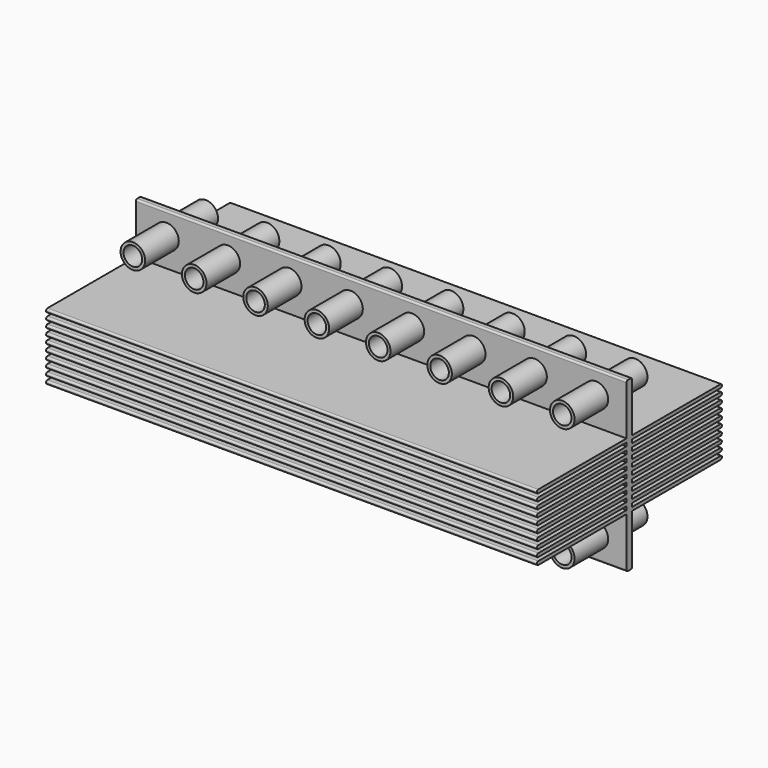
from build123d import *

# Parameters (mm, degrees)
F0_W      = 889
F0_H      = 304.8
F1_DEPTH  = 12.7
F3_D      = 33.655
F5_DEPTH  = 889
F6_R      = 3.175
F7_R      = 22.2377
F7_R_2    = 16.8275
F8_DEPTH  = 76.2
F9_R      = 22.2377
F9_R_2    = 16.8275
F10_DEPTH = 76.2


# Not quite as in the source:
# - after a boolean that leaves OpenCascade's solid faulty, fix() repairs it


with BuildPart() as f1:
    # F0 (on Front) → F1 (new body)
    with BuildSketch(Plane.XZ):
        with Locations((444.5, 152.4)):
            Rectangle(F0_W, F0_H)
    extrude(amount=F1_DEPTH)

    # F3 (through all)
    with Locations(Plane.XZ.offset(12.7)):
        with Locations((55.5752, 41.275), (55.5752, 263.5504), (166.7002, 263.5504), (166.7002, 41.275), (277.8252, 41.275), (277.8252, 263.5504), (388.9502, 263.5504), (500.0752, 41.275), (500.0752, 263.5504), (388.9502, 41.275), (611.2002, 41.275), (722.3252, 41.275), (833.4502, 41.275), (833.4502, 263.5504), (722.3252, 263.5504), (611.2002, 263.5504)):
            Hole(F3_D / 2)

    # F4 (on face) → F5 (join, through all)
    with BuildSketch(Plane(origin=(0, 0, 0), x_dir=(0, -1, 0), z_dir=(-1, 0, 0))):
        with BuildLine():
            Line((212.725, 161.925), (12.7, 161.925))
            Line((12.7, 161.925), (12.7, 155.575))
            Line((12.7, 155.575), (212.725, 155.575))
            ThreePointArc((212.725, 155.575), (214.9700640303, 156.5049359697), (215.9, 158.75))
            ThreePointArc((215.9, 158.75), (214.9700640303, 160.9950640303), (212.725, 161.925))
        make_face()
        with BuildLine():
            Line((212.725, 174.625), (12.7, 174.625))
            Line((12.7, 174.625), (12.7, 168.275))
            Line((12.7, 168.275), (212.725, 168.275))
            ThreePointArc((212.725, 168.275), (214.9700640303, 169.2049359697), (215.9, 171.45))
            ThreePointArc((215.9, 171.45), (214.9700640303, 173.6950640303), (212.725, 174.625))
        make_face()
        with BuildLine():
            Line((212.725, 187.325), (12.7, 187.325))
            Line((12.7, 187.325), (12.7, 180.975))
            Line((12.7, 180.975), (212.725, 180.975))
            ThreePointArc((212.725, 180.975), (214.9700640303, 181.9049359697), (215.9, 184.15))
            ThreePointArc((215.9, 184.15), (214.9700640303, 186.3950640303), (212.725, 187.325))
        make_face()
        with BuildLine():
            Line((212.725, 200.025), (12.7, 200.025))
            Line((12.7, 200.025), (12.7, 193.675))
            Line((12.7, 193.675), (212.725, 193.675))
            ThreePointArc((212.725, 193.675), (214.9700640303, 194.6049359697), (215.9, 196.85))
            ThreePointArc((215.9, 196.85), (214.9700640303, 199.0950640303), (212.725, 200.025))
        make_face()
        with BuildLine():
            Line((212.725, 212.725), (12.7, 212.725))
            Line((12.7, 212.725), (12.7, 206.375))
            Line((12.7, 206.375), (212.725, 206.375))
            ThreePointArc((212.725, 206.375), (214.9700640303, 207.3049359697), (215.9, 209.55))
            ThreePointArc((215.9, 209.55), (214.9700640303, 211.7950640303), (212.725, 212.725))
        make_face()
        with BuildLine():
            Line((12.7, 98.425), (12.7, 92.075))
            Line((12.7, 92.075), (212.725, 92.075))
            ThreePointArc((212.725, 92.075), (214.9700640303, 93.0049359697), (215.9, 95.25))
            ThreePointArc((215.9, 95.25), (214.9700640303, 97.4950640303), (212.725, 98.425))
            Line((212.725, 98.425), (12.7, 98.425))
        make_face()
        with BuildLine():
            Line((12.7, 111.125), (12.7, 104.775))
            Line((12.7, 104.775), (212.725, 104.775))
            ThreePointArc((212.725, 104.775), (214.9700640303, 105.7049359697), (215.9, 107.95))
            ThreePointArc((215.9, 107.95), (214.9700640303, 110.1950640303), (212.725, 111.125))
            Line((212.725, 111.125), (12.7, 111.125))
        make_face()
        with BuildLine():
            Line((12.7, 123.825), (12.7, 117.475))
            Line((12.7, 117.475), (212.725, 117.475))
            ThreePointArc((212.725, 117.475), (214.9700640303, 118.4049359697), (215.9, 120.65))
            ThreePointArc((215.9, 120.65), (214.9700640303, 122.8950640303), (212.725, 123.825))
            Line((212.725, 123.825), (12.7, 123.825))
        make_face()
        with BuildLine():
            Line((12.7, 136.525), (12.7, 130.175))
            Line((12.7, 130.175), (212.725, 130.175))
            ThreePointArc((212.725, 130.175), (214.9700640303, 131.1049359697), (215.9, 133.35))
            ThreePointArc((215.9, 133.35), (214.9700640303, 135.5950640303), (212.725, 136.525))
            Line((212.725, 136.525), (12.7, 136.525))
        make_face()
        with BuildLine():
            Line((12.7, 149.225), (12.7, 142.875))
            Line((12.7, 142.875), (212.725, 142.875))
            ThreePointArc((212.725, 142.875), (214.9700640303, 143.8049359697), (215.9, 146.05))
            ThreePointArc((215.9, 146.05), (214.9700640303, 148.2950640303), (212.725, 149.225))
            Line((212.725, 149.225), (12.7, 149.225))
        make_face()
        with BuildLine():
            Line((0, 206.375), (0, 212.725))
            Line((0, 212.725), (-200.025, 212.725))
            ThreePointArc((-200.025, 212.725), (-202.2700640303, 211.7950640303), (-203.2, 209.55))
            ThreePointArc((-203.2, 209.55), (-202.2700640303, 207.3049359697), (-200.025, 206.375))
            Line((-200.025, 206.375), (0, 206.375))
        make_face()
        with BuildLine():
            Line((0, 193.675), (0, 200.025))
            Line((0, 200.025), (-200.025, 200.025))
            ThreePointArc((-200.025, 200.025), (-202.2700640303, 199.0950640303), (-203.2, 196.85))
            ThreePointArc((-203.2, 196.85), (-202.2700640303, 194.6049359697), (-200.025, 193.675))
            Line((-200.025, 193.675), (0, 193.675))
        make_face()
        with BuildLine():
            Line((0, 180.975), (0, 187.325))
            Line((0, 187.325), (-200.025, 187.325))
            ThreePointArc((-200.025, 187.325), (-202.2700640303, 186.3950640303), (-203.2, 184.15))
            ThreePointArc((-203.2, 184.15), (-202.2700640303, 181.9049359697), (-200.025, 180.975))
            Line((-200.025, 180.975), (0, 180.975))
        make_face()
        with BuildLine():
            Line((0, 168.275), (0, 174.625))
            Line((0, 174.625), (-200.025, 174.625))
            ThreePointArc((-200.025, 174.625), (-202.2700640303, 173.6950640303), (-203.2, 171.45))
            ThreePointArc((-203.2, 171.45), (-202.2700640303, 169.2049359697), (-200.025, 168.275))
            Line((-200.025, 168.275), (0, 168.275))
        make_face()
        with BuildLine():
            Line((0, 155.575), (0, 161.925))
            Line((0, 161.925), (-200.025, 161.925))
            ThreePointArc((-200.025, 161.925), (-202.2700640303, 160.9950640303), (-203.2, 158.75))
            ThreePointArc((-203.2, 158.75), (-202.2700640303, 156.5049359697), (-200.025, 155.575))
            Line((-200.025, 155.575), (0, 155.575))
        make_face()
        with BuildLine():
            Line((-200.025, 142.875), (0, 142.875))
            Line((0, 142.875), (0, 149.225))
            Line((0, 149.225), (-200.025, 149.225))
            ThreePointArc((-200.025, 149.225), (-202.2700640303, 148.2950640303), (-203.2, 146.05))
            ThreePointArc((-203.2, 146.05), (-202.2700640303, 143.8049359697), (-200.025, 142.875))
        make_face()
        with BuildLine():
            Line((-200.025, 130.175), (0, 130.175))
            Line((0, 130.175), (0, 136.525))
            Line((0, 136.525), (-200.025, 136.525))
            ThreePointArc((-200.025, 136.525), (-202.2700640303, 135.5950640303), (-203.2, 133.35))
            ThreePointArc((-203.2, 133.35), (-202.2700640303, 131.1049359697), (-200.025, 130.175))
        make_face()
        with BuildLine():
            Line((-200.025, 117.475), (0, 117.475))
            Line((0, 117.475), (0, 123.825))
            Line((0, 123.825), (-200.025, 123.825))
            ThreePointArc((-200.025, 123.825), (-202.2700640303, 122.8950640303), (-203.2, 120.65))
            ThreePointArc((-203.2, 120.65), (-202.2700640303, 118.4049359697), (-200.025, 117.475))
        make_face()
        with BuildLine():
            Line((-200.025, 104.775), (0, 104.775))
            Line((0, 104.775), (0, 111.125))
            Line((0, 111.125), (-200.025, 111.125))
            ThreePointArc((-200.025, 111.125), (-202.2700640303, 110.1950640303), (-203.2, 107.95))
            ThreePointArc((-203.2, 107.95), (-202.2700640303, 105.7049359697), (-200.025, 104.775))
        make_face()
        with BuildLine():
            Line((-200.025, 92.075), (0, 92.075))
            Line((0, 92.075), (0, 98.425))
            Line((0, 98.425), (-200.025, 98.425))
            ThreePointArc((-200.025, 98.425), (-202.2700640303, 97.4950640303), (-203.2, 95.25))
            ThreePointArc((-203.2, 95.25), (-202.2700640303, 93.0049359697), (-200.025, 92.075))
        make_face()
    extrude(amount=-F5_DEPTH)

    # F6
    f6_edges = [f1.edges().sort_by_distance(p)[0] for p in [
        (444.5, 0, 0),
        (444.5, -12.7, 0),
        (444.5, -12.7, 304.8),
        (444.5, 0, 304.8),
    ]]
    fillet(f6_edges, radius=F6_R)

    # F7 (on face) → F8 (join)
    with BuildSketch(Plane(origin=(0, 0, 0), x_dir=(-1, 0, 0), z_dir=(0, 1, 0))):
        with Locations((-55.5752, 41.275)):
            Circle(F7_R)
        with Locations((-55.5752, 41.275)):
            Circle(F7_R_2, mode=Mode.SUBTRACT)
        with Locations((-55.5752, 263.5504)):
            Circle(F7_R)
        with Locations((-55.5752, 263.5504)):
            Circle(F7_R_2, mode=Mode.SUBTRACT)
        with Locations((-166.7002, 41.275)):
            Circle(F7_R)
        with Locations((-166.7002, 41.275)):
            Circle(F7_R_2, mode=Mode.SUBTRACT)
        with Locations((-166.7002, 263.5504)):
            Circle(F7_R)
        with Locations((-166.7002, 263.5504)):
            Circle(F7_R_2, mode=Mode.SUBTRACT)
        with Locations((-277.8252, 41.275)):
            Circle(F7_R)
        with Locations((-277.8252, 41.275)):
            Circle(F7_R_2, mode=Mode.SUBTRACT)
        with Locations((-277.8252, 263.5504)):
            Circle(F7_R)
        with Locations((-277.8252, 263.5504)):
            Circle(F7_R_2, mode=Mode.SUBTRACT)
        with Locations((-388.9502, 41.275)):
            Circle(F7_R)
        with Locations((-388.9502, 41.275)):
            Circle(F7_R_2, mode=Mode.SUBTRACT)
        with Locations((-388.9502, 263.5504)):
            Circle(F7_R)
        with Locations((-388.9502, 263.5504)):
            Circle(F7_R_2, mode=Mode.SUBTRACT)
        with Locations((-500.0752, 41.275)):
            Circle(F7_R)
        with Locations((-500.0752, 41.275)):
            Circle(F7_R_2, mode=Mode.SUBTRACT)
        with Locations((-500.0752, 263.5504)):
            Circle(F7_R)
        with Locations((-500.0752, 263.5504)):
            Circle(F7_R_2, mode=Mode.SUBTRACT)
        with Locations((-611.2002, 41.275)):
            Circle(F7_R)
        with Locations((-611.2002, 41.275)):
            Circle(F7_R_2, mode=Mode.SUBTRACT)
        with Locations((-611.2002, 263.5504)):
            Circle(F7_R)
        with Locations((-611.2002, 263.5504)):
            Circle(F7_R_2, mode=Mode.SUBTRACT)
        with Locations((-722.3252, 41.275)):
            Circle(F7_R)
        with Locations((-722.3252, 41.275)):
            Circle(F7_R_2, mode=Mode.SUBTRACT)
        with Locations((-722.3252, 263.5504)):
            Circle(F7_R)
        with Locations((-722.3252, 263.5504)):
            Circle(F7_R_2, mode=Mode.SUBTRACT)
        with Locations((-833.4502, 41.275)):
            Circle(F7_R)
        with Locations((-833.4502, 41.275)):
            Circle(F7_R_2, mode=Mode.SUBTRACT)
        with Locations((-833.4502, 263.5504)):
            Circle(F7_R)
        with Locations((-833.4502, 263.5504)):
            Circle(F7_R_2, mode=Mode.SUBTRACT)
    extrude(amount=F8_DEPTH)

    # F9 (on face) → F10 (join)
    with BuildSketch(Plane.XZ.offset(12.7)):
        with Locations((55.5752, 41.275)):
            Circle(F9_R)
        with Locations((55.5752, 41.275)):
            Circle(F9_R_2, mode=Mode.SUBTRACT)
        with Locations((55.5752, 263.5504)):
            Circle(F9_R)
        with Locations((55.5752, 263.5504)):
            Circle(F9_R_2, mode=Mode.SUBTRACT)
        with Locations((166.7002, 41.275)):
            Circle(F9_R)
        with Locations((166.7002, 41.275)):
            Circle(F9_R_2, mode=Mode.SUBTRACT)
        with Locations((166.7002, 263.5504)):
            Circle(F9_R)
        with Locations((166.7002, 263.5504)):
            Circle(F9_R_2, mode=Mode.SUBTRACT)
        with Locations((277.8252, 41.275)):
            Circle(F9_R)
        with Locations((277.8252, 41.275)):
            Circle(F9_R_2, mode=Mode.SUBTRACT)
        with Locations((277.8252, 263.5504)):
            Circle(F9_R)
        with Locations((277.8252, 263.5504)):
            Circle(F9_R_2, mode=Mode.SUBTRACT)
        with Locations((388.9502, 41.275)):
            Circle(F9_R)
        with Locations((388.9502, 41.275)):
            Circle(F9_R_2, mode=Mode.SUBTRACT)
        with Locations((388.9502, 263.5504)):
            Circle(F9_R)
        with Locations((388.9502, 263.5504)):
            Circle(F9_R_2, mode=Mode.SUBTRACT)
        with Locations((500.0752, 41.275)):
            Circle(F9_R)
        with Locations((500.0752, 41.275)):
            Circle(F9_R_2, mode=Mode.SUBTRACT)
        with Locations((500.0752, 263.5504)):
            Circle(F9_R)
        with Locations((500.0752, 263.5504)):
            Circle(F9_R_2, mode=Mode.SUBTRACT)
        with Locations((611.2002, 41.275)):
            Circle(F9_R)
        with Locations((611.2002, 41.275)):
            Circle(F9_R_2, mode=Mode.SUBTRACT)
        with Locations((611.2002, 263.5504)):
            Circle(F9_R)
        with Locations((611.2002, 263.5504)):
            Circle(F9_R_2, mode=Mode.SUBTRACT)
        with Locations((722.3252, 41.275)):
            Circle(F9_R)
        with Locations((722.3252, 41.275)):
            Circle(F9_R_2, mode=Mode.SUBTRACT)
        with Locations((722.3252, 263.5504)):
            Circle(F9_R)
        with Locations((722.3252, 263.5504)):
            Circle(F9_R_2, mode=Mode.SUBTRACT)
        with Locations((833.4502, 41.275)):
            Circle(F9_R)
        with Locations((833.4502, 41.275)):
            Circle(F9_R_2, mode=Mode.SUBTRACT)
        with Locations((833.4502, 263.5504)):
            Circle(F9_R)
        with Locations((833.4502, 263.5504)):
            Circle(F9_R_2, mode=Mode.SUBTRACT)
    extrude(amount=F10_DEPTH)

    add(f1.part.fix(), mode=Mode.REPLACE)


solid = f1.part
